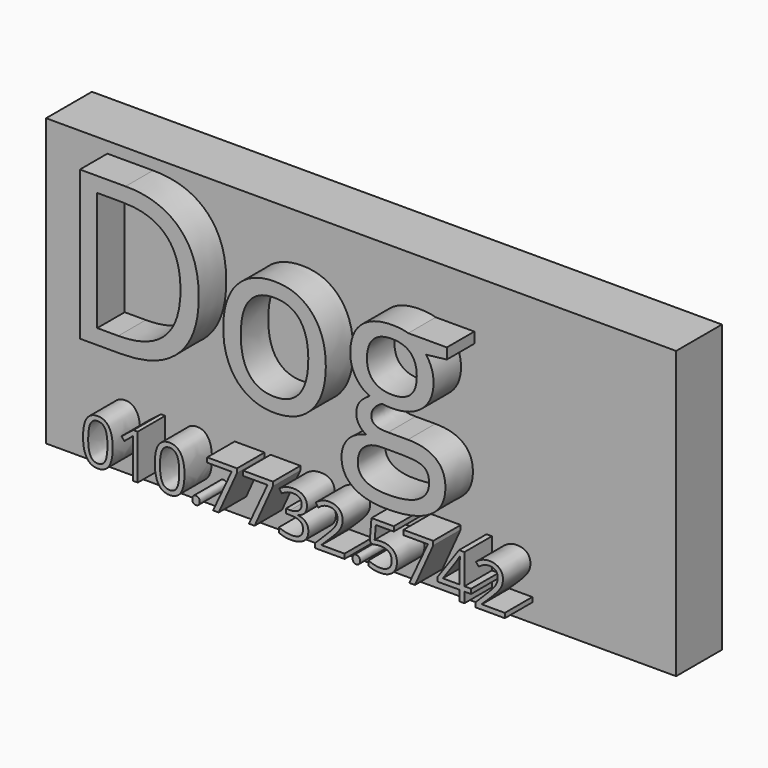
from build123d import *

# Parameters (mm, degrees)
F0_W         = 55
F0_H         = 25
F1_DEPTH     = 5
F2_TEXT_SIZE = 18.2113821138
F3_DEPTH     = 3
F4_TEXT_SIZE = 5.4818025092
F5_DEPTH     = 3


# Not quite as in the source:
# - Text() gives the source's letters only with a copy of the font that has no kerning and outlines rounded to 1/6400 em; it was checked with that copy


with BuildPart() as f1:
    # F0 (on Front) → F1 (new body)
    with BuildSketch(Plane.XZ):
        with Locations((27.5, 12.5)):
            Rectangle(F0_W, F0_H)
    extrude(amount=F1_DEPTH)

    # F2 (on face) → F3 (join)
    with BuildSketch(Plane.XZ.offset(5)):
        with Locations((3.5655973391, 11.016858047)):
            Text('Dog', F2_TEXT_SIZE, font='Open Sans', text_align=(TextAlign.LEFT, TextAlign.BOTTOM))
    extrude(amount=F3_DEPTH)

    # F4 (on face) → F5 (join)
    with BuildSketch(Plane.XZ.offset(5)):
        with Locations((5.352589209, 1.5975537244)):
            Text('010.7732.5742', F4_TEXT_SIZE, font='Open Sans', text_align=(TextAlign.LEFT, TextAlign.BOTTOM))
    extrude(amount=F5_DEPTH)


solid = f1.part
